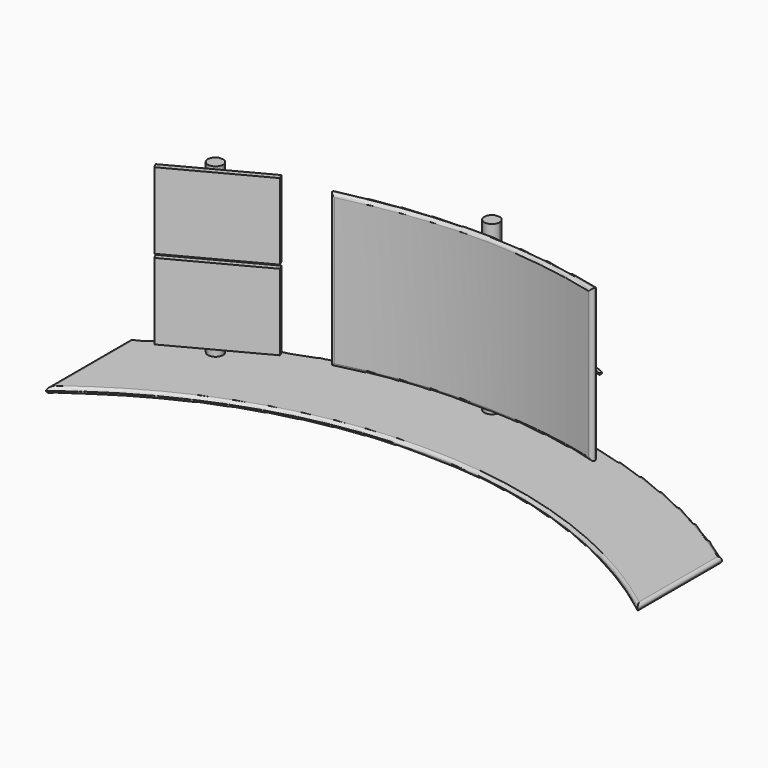
from build123d import *

# Parameters (mm, degrees)
F0_R         = 0.635
F1_DEPTH     = 0.508
F2_R         = 0.25399
F3_DEPTH     = 12.7
F5_DEPTH     = 6.35
F8_DEPTH     = 13.97
F9_DEPTH     = 1.016
F10_DEPTH    = 0.5969
F16_R        = 0.254
F19_T1_DEPTH = 13.6911805715
F19_T3_DEPTH = 13.6871611944
F19_T6_ANGLE = 30.5932209567
F19_T8_ANGLE = 30.5932209567
F20_DEPTH    = 0.127


# Not quite as in the source:
# - a fillet or chamfer that OpenCascade refuses, or shapes differently, is made with other operations: its cross-section is extruded or revolved along the edge and cut away or added
# - a fillet or chamfer is up to 0.001 mm smaller than in the source, because OpenCascade refuses the exact size


with BuildPart() as f1:
    # F0 (on Top) → F1 (new body)
    with BuildSketch(Plane.XY):
        with BuildLine():
            Line((24.6418640018, -8.8223936036), (24.6418640018, 0))
            ThreePointArc((24.6418640018, 0), (0, 7.9108268994), (-24.6418640018, 0))
            Line((-24.6418640018, 0), (-24.6418640018, -8.8223936036))
            ThreePointArc((-24.6418640018, -8.8223936036), (0, -0.2979005565), (24.6418640018, -8.8223936036))
        make_face()
        Polygon((-22.0129160094, -0.702014463), (-14.64919094, 3.2156321686), (-14.4481033974, 2.8160840178), (-21.8028810519, -1.096802413), align=None, mode=Mode.SUBTRACT)
        with Locations((-19.1195905209, 1.9358670106)):
            Circle(F0_R, mode=Mode.SUBTRACT)
        with BuildLine():
            ThreePointArc((-10.9774693847, 4.2001847178), (-0.0735459077, 5.6055651856), (10.8358133584, 4.2430227622))
            Line((10.8358133584, 4.2430227622), (10.8358133584, 3.6900111008))
            ThreePointArc((10.8358133584, 3.6900111008), (-0.073155619, 5.0882435822), (-10.9774693847, 3.6541586742))
            Line((-10.9774693847, 3.6541586742), (-10.9774693847, 4.2001847178))
        make_face(mode=Mode.SUBTRACT)
        with BuildLine():
            ThreePointArc((0.2075697848, 7.5781678897), (0.3505706678, 7.5220443298), (0.4795346964, 7.4385734616))
            ThreePointArc((0.4795346964, 7.4385734616), (5.6853396024, 6.773279999), (10.6270741671, 5.006282658))
            Line((10.6270741671, 5.006282658), (10.6270741671, 4.752282658))
            ThreePointArc((10.6270741671, 4.752282658), (5.7883534557, 6.2215479995), (0.7675825056, 6.8247211363))
            ThreePointArc((0.7675825056, 6.8247211363), (-0.0041251816, 6.0713398006), (-0.767692111, 6.8329707714))
            ThreePointArc((-0.767692111, 6.8329707714), (-5.8505234125, 6.272612966), (-10.7549736276, 4.8250139203))
            Line((-10.7549736276, 4.8250139203), (-10.7549736276, 4.9255372574))
            ThreePointArc((-10.7549736276, 4.9255372574), (-5.7560035668, 6.7472117335), (-0.4804700318, 7.437824133))
            ThreePointArc((-0.4804700318, 7.437824133), (-0.3531560296, 7.5207111182), (-0.2120132338, 7.5769055903))
            Line((-0.2120132338, 7.5769055903), (-0.2120132338, 7.6930532232))
            Line((-0.2120132338, 7.6930532232), (0.2075697848, 7.6930532232))
            Line((0.2075697848, 7.6930532232), (0.2075697848, 7.5781678897))
        make_face(mode=Mode.SUBTRACT)
        with Locations((18.3151047677, 1.9358670106)):
            Circle(F0_R, mode=Mode.SUBTRACT)
        with BuildLine():
            Line((10.8358133584, 3.6900111008), (10.8358133584, 4.2430227622))
            ThreePointArc((10.8358133584, 4.2430227622), (-0.0735459077, 5.6055651856), (-10.9774693847, 4.2001847178))
            Line((-10.9774693847, 4.2001847178), (-10.9774693847, 3.6541586742))
            ThreePointArc((-10.9774693847, 3.6541586742), (-0.073155619, 5.0882435822), (10.8358133584, 3.6900111008))
        make_face()
        with BuildLine():
            ThreePointArc((10.6270741671, 5.006282658), (5.6853396024, 6.773279999), (0.4795346964, 7.4385734616))
            ThreePointArc((0.4795346964, 7.4385734616), (0.6919301258, 7.1716418705), (0.7677161402, 6.8390448578))
            ThreePointArc((0.7677161402, 6.8390448578), (0.7676827308, 6.8318826853), (0.7675825056, 6.8247211363))
            ThreePointArc((0.7675825056, 6.8247211363), (5.7883534557, 6.2215479995), (10.6270741671, 4.752282658))
            Line((10.6270741671, 4.752282658), (10.6270741671, 5.006282658))
        make_face()
        with BuildLine():
            ThreePointArc((-0.767692111, 6.8329707714), (-0.6934977152, 7.1683608017), (-0.4804700318, 7.437824133))
            ThreePointArc((-0.4804700318, 7.437824133), (-5.7560035668, 6.7472117335), (-10.7549736276, 4.9255372574))
            Line((-10.7549736276, 4.9255372574), (-10.7549736276, 4.8250139203))
            ThreePointArc((-10.7549736276, 4.8250139203), (-5.8505234125, 6.272612966), (-0.767692111, 6.8329707714))
        make_face()
        Polygon((-14.4481033974, 2.8160840178), (-14.64919094, 3.2156321686), (-22.0129160094, -0.702014463), (-21.8028810519, -1.096802413), align=None)
        with Locations((-19.1195905209, 1.9358670106)):
            Circle(F0_R)
        with Locations((18.3151047677, 1.9358670106)):
            Circle(F0_R)
        with BuildLine():
            ThreePointArc((-0.634989989, 6.8354792114), (-0.0034120558, 6.2040540249), (0.6349150034, 6.8286555117))
            ThreePointArc((0.6349150034, 6.8286555117), (0, 6.8390448578), (-0.634989989, 6.8354792114))
        make_face()
        with BuildLine():
            ThreePointArc((0.6349150034, 6.8286555117), (0.6349787505, 6.8338500109), (0.635, 6.8390448578))
            ThreePointArc((0.635, 6.8390448578), (0.5143735851, 7.2113952505), (0.1983234175, 7.4422801535))
            ThreePointArc((0.1983234175, 7.4422801535), (-0.0004713667, 7.4429377567), (-0.1992648821, 7.4419698173))
            ThreePointArc((-0.1992648821, 7.4419698173), (-0.5157063227, 7.2095472043), (-0.634989989, 6.8354792114))
            ThreePointArc((-0.634989989, 6.8354792114), (0, 6.8390448578), (0.6349150034, 6.8286555117))
        make_face()
        with BuildLine():
            ThreePointArc((0.7675825056, 6.8247211363), (0.7012510135, 6.8267645002), (0.6349150034, 6.8286555117))
            ThreePointArc((0.6349150034, 6.8286555117), (-0.0034120558, 6.2040540249), (-0.634989989, 6.8354792114))
            ThreePointArc((-0.634989989, 6.8354792114), (-0.7013424903, 6.8343011875), (-0.767692111, 6.8329707714))
            ThreePointArc((-0.767692111, 6.8329707714), (-0.0041251816, 6.0713398006), (0.7675825056, 6.8247211363))
        make_face()
        with BuildLine():
            ThreePointArc((0.1983234175, 7.4422801535), (0.5143735851, 7.2113952505), (0.635, 6.8390448578))
            ThreePointArc((0.635, 6.8390448578), (0.6349787505, 6.8338500109), (0.6349150034, 6.8286555117))
            ThreePointArc((0.6349150034, 6.8286555117), (0.7012510135, 6.8267645002), (0.7675825056, 6.8247211363))
            ThreePointArc((0.7675825056, 6.8247211363), (0.7676827308, 6.8318826853), (0.7677161402, 6.8390448578))
            ThreePointArc((0.7677161402, 6.8390448578), (0.6919301258, 7.1716418705), (0.4795346964, 7.4385734616))
            ThreePointArc((0.4795346964, 7.4385734616), (0.3389344168, 7.4408334387), (0.1983234175, 7.4422801535))
        make_face()
        with BuildLine():
            ThreePointArc((-0.634989989, 6.8354792114), (-0.5157063227, 7.2095472043), (-0.1992648821, 7.4419698173))
            ThreePointArc((-0.1992648821, 7.4419698173), (-0.3398734516, 7.4403035974), (-0.4804700318, 7.437824133))
            ThreePointArc((-0.4804700318, 7.437824133), (-0.6934977152, 7.1683608017), (-0.767692111, 6.8329707714))
            ThreePointArc((-0.767692111, 6.8329707714), (-0.7013424903, 6.8343011875), (-0.634989989, 6.8354792114))
        make_face()
        with BuildLine():
            ThreePointArc((-0.1992648821, 7.4419698173), (-0.0004956471, 7.4740446643), (0.1983234175, 7.4422801535))
            ThreePointArc((0.1983234175, 7.4422801535), (0.3389344168, 7.4408334387), (0.4795346964, 7.4385734616))
            ThreePointArc((0.4795346964, 7.4385734616), (0.3505706678, 7.5220443298), (0.2075697848, 7.5781678897))
            Line((0.2075697848, 7.5781678897), (0.2075697848, 7.5769055903))
            Line((0.2075697848, 7.5769055903), (-0.2120132338, 7.5769055903))
            ThreePointArc((-0.2120132338, 7.5769055903), (-0.3531560296, 7.5207111182), (-0.4804700318, 7.437824133))
            ThreePointArc((-0.4804700318, 7.437824133), (-0.3398734516, 7.4403035974), (-0.1992648821, 7.4419698173))
        make_face()
        with BuildLine():
            ThreePointArc((-0.2120132338, 7.5769055903), (-0.0023096341, 7.6067575237), (0.2075697848, 7.5781678897))
            Line((0.2075697848, 7.5781678897), (0.2075697848, 7.6930532232))
            Line((0.2075697848, 7.6930532232), (-0.2120132338, 7.6930532232))
            Line((-0.2120132338, 7.6930532232), (-0.2120132338, 7.5769055903))
        make_face()
        with BuildLine():
            Line((0.2075697848, 7.5769055903), (0.2075697848, 7.5781678897))
            ThreePointArc((0.2075697848, 7.5781678897), (-0.0023096341, 7.6067575237), (-0.2120132338, 7.5769055903))
            Line((-0.2120132338, 7.5769055903), (0.2075697848, 7.5769055903))
        make_face()
        with BuildLine():
            ThreePointArc((-0.1992648821, 7.4419698173), (-0.0004713667, 7.4429377567), (0.1983234175, 7.4422801535))
            ThreePointArc((0.1983234175, 7.4422801535), (-0.0004956471, 7.4740446643), (-0.1992648821, 7.4419698173))
        make_face()
    extrude(amount=-F1_DEPTH)

    # F2 (radius 0.254 in the source; OpenCascade refuses exactly that, so slightly less here)
    f2_edges = [f1.edges().sort_by_distance(p)[0] for p in [
        (0, -0.297901, 0),
        (24.641864, -4.411197, 0),
        (0, 7.910827, 0),
        (-24.641864, -4.411197, 0),
        (0, -0.297901, -0.508),
        (24.641864, -4.411197, -0.508),
        (0, 7.910827, -0.508),
        (-24.641864, -4.411197, -0.508),
    ]]
    fillet(f2_edges, radius=F2_R)


with BuildPart() as f3:
    # F0 (on Top) → F3 (new body)
    with BuildSketch(Plane.XY):
        with BuildLine():
            Line((10.8358133584, 3.6900111008), (10.8358133584, 4.2430227622))
            ThreePointArc((10.8358133584, 4.2430227622), (-0.0735459077, 5.6055651856), (-10.9774693847, 4.2001847178))
            Line((-10.9774693847, 4.2001847178), (-10.9774693847, 3.6541586742))
            ThreePointArc((-10.9774693847, 3.6541586742), (-0.073155619, 5.0882435822), (10.8358133584, 3.6900111008))
        make_face()
    extrude(amount=F3_DEPTH)


with BuildPart() as f3_1:
    # F4: moved
    add(f3.part.moved(Location((0, 0, 0.9398))))

    # F16
    f16_edges = [f3_1.edges().sort_by_distance(p)[0] for p in [
        (-10.977469, 3.654159, 7.2898),
        (10.835813, 3.690011, 7.2898),
        (-0.073156, 5.088244, 0.9398),
        (-0.073156, 5.088244, 13.6398),
    ]]
    fillet(f16_edges, radius=F16_R)


with BuildPart() as f5:
    # F0 (on Top) → F5 (new body)
    with BuildSketch(Plane.XY):
        Polygon((-14.4481033974, 2.8160840178), (-14.64919094, 3.2156321686), (-22.0129160094, -0.702014463), (-21.8028810519, -1.096802413), align=None)
    extrude(amount=F5_DEPTH)


with BuildPart() as f5_1:
    # F6: moved
    add(f5.part.moved(Location((0, 0, 0.9398))))


with BuildPart() as f7_1:
    # F7: copy of F5
    add(f5_1.part.moved(Location((0, 0, 6.6548))))


with BuildPart() as f8:
    # F0 (on Top) → F8 (new body)
    with BuildSketch(Plane.XY):
        with BuildLine():
            ThreePointArc((-0.634989989, 6.8354792114), (-0.0034120558, 6.2040540249), (0.6349150034, 6.8286555117))
            ThreePointArc((0.6349150034, 6.8286555117), (0, 6.8390448578), (-0.634989989, 6.8354792114))
        make_face()
        with BuildLine():
            ThreePointArc((0.6349150034, 6.8286555117), (0.6349787505, 6.8338500109), (0.635, 6.8390448578))
            ThreePointArc((0.635, 6.8390448578), (0.5143735851, 7.2113952505), (0.1983234175, 7.4422801535))
            ThreePointArc((0.1983234175, 7.4422801535), (-0.0004713667, 7.4429377567), (-0.1992648821, 7.4419698173))
            ThreePointArc((-0.1992648821, 7.4419698173), (-0.5157063227, 7.2095472043), (-0.634989989, 6.8354792114))
            ThreePointArc((-0.634989989, 6.8354792114), (0, 6.8390448578), (0.6349150034, 6.8286555117))
        make_face()
    extrude(amount=F8_DEPTH)


with BuildPart() as f9:
    # F0 (on Top) → F9 (new body)
    with BuildSketch(Plane.XY):
        with BuildLine():
            ThreePointArc((0.7675825056, 6.8247211363), (0.7012510135, 6.8267645002), (0.6349150034, 6.8286555117))
            ThreePointArc((0.6349150034, 6.8286555117), (-0.0034120558, 6.2040540249), (-0.634989989, 6.8354792114))
            ThreePointArc((-0.634989989, 6.8354792114), (-0.7013424903, 6.8343011875), (-0.767692111, 6.8329707714))
            ThreePointArc((-0.767692111, 6.8329707714), (-0.0041251816, 6.0713398006), (0.7675825056, 6.8247211363))
        make_face()
        with BuildLine():
            ThreePointArc((-0.634989989, 6.8354792114), (-0.5157063227, 7.2095472043), (-0.1992648821, 7.4419698173))
            ThreePointArc((-0.1992648821, 7.4419698173), (-0.3398734516, 7.4403035974), (-0.4804700318, 7.437824133))
            ThreePointArc((-0.4804700318, 7.437824133), (-0.6934977152, 7.1683608017), (-0.767692111, 6.8329707714))
            ThreePointArc((-0.767692111, 6.8329707714), (-0.7013424903, 6.8343011875), (-0.634989989, 6.8354792114))
        make_face()
        with BuildLine():
            ThreePointArc((0.1983234175, 7.4422801535), (0.5143735851, 7.2113952505), (0.635, 6.8390448578))
            ThreePointArc((0.635, 6.8390448578), (0.6349787505, 6.8338500109), (0.6349150034, 6.8286555117))
            ThreePointArc((0.6349150034, 6.8286555117), (0.7012510135, 6.8267645002), (0.7675825056, 6.8247211363))
            ThreePointArc((0.7675825056, 6.8247211363), (0.7676827308, 6.8318826853), (0.7677161402, 6.8390448578))
            ThreePointArc((0.7677161402, 6.8390448578), (0.6919301258, 7.1716418705), (0.4795346964, 7.4385734616))
            ThreePointArc((0.4795346964, 7.4385734616), (0.3389344168, 7.4408334387), (0.1983234175, 7.4422801535))
        make_face()
        with BuildLine():
            ThreePointArc((-0.1992648821, 7.4419698173), (-0.0004956471, 7.4740446643), (0.1983234175, 7.4422801535))
            ThreePointArc((0.1983234175, 7.4422801535), (0.3389344168, 7.4408334387), (0.4795346964, 7.4385734616))
            ThreePointArc((0.4795346964, 7.4385734616), (0.3505706678, 7.5220443298), (0.2075697848, 7.5781678897))
            Line((0.2075697848, 7.5781678897), (0.2075697848, 7.5769055903))
            Line((0.2075697848, 7.5769055903), (-0.2120132338, 7.5769055903))
            ThreePointArc((-0.2120132338, 7.5769055903), (-0.3531560296, 7.5207111182), (-0.4804700318, 7.437824133))
            ThreePointArc((-0.4804700318, 7.437824133), (-0.3398734516, 7.4403035974), (-0.1992648821, 7.4419698173))
        make_face()
    extrude(amount=F9_DEPTH)


with BuildPart() as f10:
    # F0 (on Top) → F10 (new body)
    with BuildSketch(Plane.XY):
        with BuildLine():
            ThreePointArc((-0.2120132338, 7.5769055903), (-0.0023096341, 7.6067575237), (0.2075697848, 7.5781678897))
            Line((0.2075697848, 7.5781678897), (0.2075697848, 7.6930532232))
            Line((0.2075697848, 7.6930532232), (-0.2120132338, 7.6930532232))
            Line((-0.2120132338, 7.6930532232), (-0.2120132338, 7.5769055903))
        make_face()
        with BuildLine():
            Line((0.2075697848, 7.5769055903), (0.2075697848, 7.5781678897))
            ThreePointArc((0.2075697848, 7.5781678897), (-0.0023096341, 7.6067575237), (-0.2120132338, 7.5769055903))
            Line((-0.2120132338, 7.5769055903), (0.2075697848, 7.5769055903))
        make_face()
    extrude(amount=F10_DEPTH)


with BuildPart() as f10_1:
    # F11: moved
    add(f10.part.moved(Location((0, 0, 0.18796))))


with BuildPart() as f10_2:
    # F12: moved
    add(f10_1.part.moved(Location((0, 0, 6.4262))))


with BuildPart() as f9_1:
    # F12: moved
    add(f9.part.moved(Location((0, 0, 6.4262))))


with BuildPart() as f13_1:
    # F13: copy of F8
    add(f8.part.moved(Location((-19.1262, -4.9022, 0))))


with BuildPart() as f14_1:
    # F14: copy of F9
    add(f9_1.part.moved(Location((-19.1262, -4.9022, 0))))


with BuildPart() as f15_1:
    # F15: copy of F10
    add(f10_2.part.moved(Location((-19.11604, -4.90982, 0))))


with BuildPart() as f17_1:
    # F17: copy of F3
    add(f3_1.part)


with BuildPart() as f3_2:
    add(f3_1.part)

    # F19: fillet of radius 0.254 on 4 edges, made by hand

    # F19_s2 → F19_t1 (cut)
    with BuildSketch(Plane.XY.offset(0.4442097143)):
        with BuildLine():
            ThreePointArc((10.6436519813, 4.2917214497), (10.7820919272, 4.2015833975), (10.8358133584, 4.0453640169))
            Line((10.8358133584, 4.0453640169), (10.8358133584, 4.2430227622))
            ThreePointArc((10.8358133584, 4.2430227622), (10.7397603039, 4.2674811479), (10.6436519813, 4.2917214497))
        make_face()
    extrude(amount=F19_T1_DEPTH, mode=Mode.SUBTRACT)

    # F19_s4 → F19_t3 (cut)
    with BuildSketch(Plane.XY.offset(0.4462194028)):
        with BuildLine():
            ThreePointArc((-10.9774693847, 4.0033275065), (-10.9240557925, 4.1591514231), (-10.7862796762, 4.2494390001))
            ThreePointArc((-10.7862796762, 4.2494390001), (-10.8819023664, 4.2249199095), (-10.9774693847, 4.2001847178))
            Line((-10.9774693847, 4.2001847178), (-10.9774693847, 4.0033275065))
        make_face()
    extrude(amount=F19_T3_DEPTH, mode=Mode.SUBTRACT)

    # F19_s5 → F19_t6 (revolve, cut)
    with BuildSketch(Plane(origin=(9.6327426049, -2.6142862112, 0), x_dir=(0, 0, 1), z_dir=(0.9650892614, -0.2619212048, 0))):
        with BuildLine():
            ThreePointArc((0.9398, -6.6836422058), (1.0141948776, -6.8632473283), (1.1938, -6.9376422058))
            Line((1.1938, -6.9376422058), (0.9398, -6.9376422058))
            Line((0.9398, -6.9376422058), (0.9398, -6.6836422058))
        make_face()
    revolve(axis=Axis((0.0122119204, -38.0626221314, 0.9398), (0, 0, 1)), revolution_arc=F19_T6_ANGLE, mode=Mode.SUBTRACT)

    # F19_s7 → F19_t8 (revolve, cut)
    with BuildSketch(Plane(origin=(9.6327426049, -2.6142862112, 0), x_dir=(0, 0, 1), z_dir=(0.9650892614, -0.2619212048, 0))):
        with BuildLine():
            ThreePointArc((13.3858, -6.9376422058), (13.5654051224, -6.8632473283), (13.6398, -6.6836422058))
            Line((13.6398, -6.6836422058), (13.6398, -6.9376422058))
            Line((13.6398, -6.9376422058), (13.3858, -6.9376422058))
        make_face()
    revolve(axis=Axis((0.0122119204, -38.0626221314, 13.6398), (0, 0, 1)), revolution_arc=F19_T8_ANGLE, mode=Mode.SUBTRACT)


with BuildPart() as f20:
    # F0 (on Top) → F20 (new body)
    with BuildSketch(Plane.XY):
        with BuildLine():
            ThreePointArc((10.6270741671, 5.006282658), (5.6853396024, 6.773279999), (0.4795346964, 7.4385734616))
            ThreePointArc((0.4795346964, 7.4385734616), (0.6919301258, 7.1716418705), (0.7677161402, 6.8390448578))
            ThreePointArc((0.7677161402, 6.8390448578), (0.7676827308, 6.8318826853), (0.7675825056, 6.8247211363))
            ThreePointArc((0.7675825056, 6.8247211363), (5.7883534557, 6.2215479995), (10.6270741671, 4.752282658))
            Line((10.6270741671, 4.752282658), (10.6270741671, 5.006282658))
        make_face()
        with BuildLine():
            ThreePointArc((-0.767692111, 6.8329707714), (-0.6934977152, 7.1683608017), (-0.4804700318, 7.437824133))
            ThreePointArc((-0.4804700318, 7.437824133), (-5.7560035668, 6.7472117335), (-10.7549736276, 4.9255372574))
            Line((-10.7549736276, 4.9255372574), (-10.7549736276, 4.8250139203))
            ThreePointArc((-10.7549736276, 4.8250139203), (-5.8505234125, 6.272612966), (-0.767692111, 6.8329707714))
        make_face()
        with BuildLine():
            ThreePointArc((0.6349150034, 6.8286555117), (0.6349787505, 6.8338500109), (0.635, 6.8390448578))
            ThreePointArc((0.635, 6.8390448578), (0.5143735851, 7.2113952505), (0.1983234175, 7.4422801535))
            ThreePointArc((0.1983234175, 7.4422801535), (-0.0004713667, 7.4429377567), (-0.1992648821, 7.4419698173))
            ThreePointArc((-0.1992648821, 7.4419698173), (-0.5157063227, 7.2095472043), (-0.634989989, 6.8354792114))
            ThreePointArc((-0.634989989, 6.8354792114), (0, 6.8390448578), (0.6349150034, 6.8286555117))
        make_face()
        with BuildLine():
            ThreePointArc((0.1983234175, 7.4422801535), (0.5143735851, 7.2113952505), (0.635, 6.8390448578))
            ThreePointArc((0.635, 6.8390448578), (0.6349787505, 6.8338500109), (0.6349150034, 6.8286555117))
            ThreePointArc((0.6349150034, 6.8286555117), (0.7012510135, 6.8267645002), (0.7675825056, 6.8247211363))
            ThreePointArc((0.7675825056, 6.8247211363), (0.7676827308, 6.8318826853), (0.7677161402, 6.8390448578))
            ThreePointArc((0.7677161402, 6.8390448578), (0.6919301258, 7.1716418705), (0.4795346964, 7.4385734616))
            ThreePointArc((0.4795346964, 7.4385734616), (0.3389344168, 7.4408334387), (0.1983234175, 7.4422801535))
        make_face()
        with BuildLine():
            ThreePointArc((-0.634989989, 6.8354792114), (-0.5157063227, 7.2095472043), (-0.1992648821, 7.4419698173))
            ThreePointArc((-0.1992648821, 7.4419698173), (-0.3398734516, 7.4403035974), (-0.4804700318, 7.437824133))
            ThreePointArc((-0.4804700318, 7.437824133), (-0.6934977152, 7.1683608017), (-0.767692111, 6.8329707714))
            ThreePointArc((-0.767692111, 6.8329707714), (-0.7013424903, 6.8343011875), (-0.634989989, 6.8354792114))
        make_face()
    extrude(amount=F20_DEPTH)


with BuildPart() as f20_1:
    # F21: moved
    add(f20.part.moved(Location((0, 0, 6.858))))


solid = Compound([f1.part, f5_1.part, f7_1.part, f8.part, f10_2.part, f9_1.part, f13_1.part, f14_1.part, f15_1.part, f3_2.part, f20_1.part])
